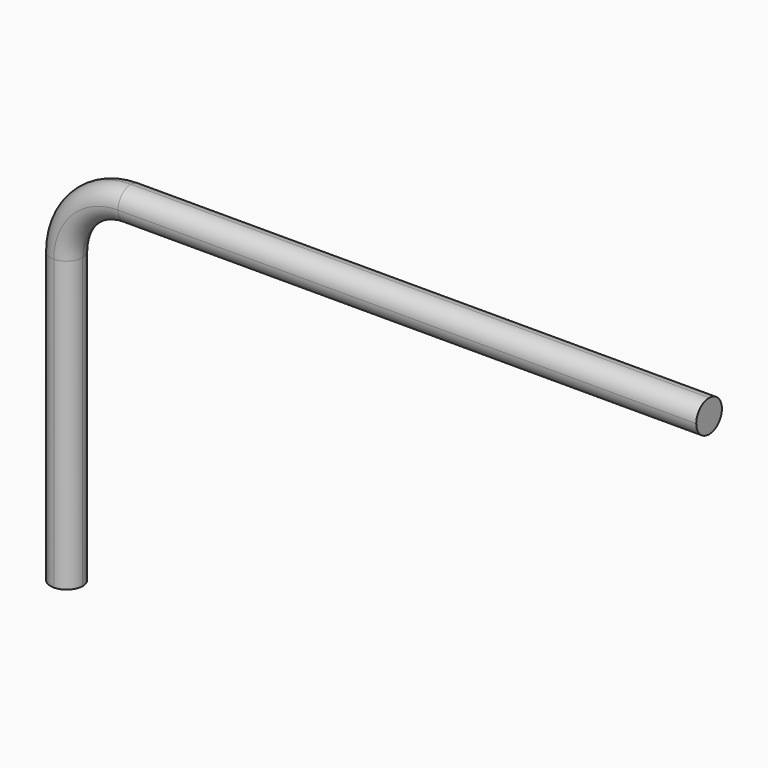
from build123d import *

# Parameters (mm, degrees)
F1_DEPTH = 25.4
F2_R     = 25.39999


# Not quite as in the source:
# - a fillet or chamfer is up to 0.001 mm smaller than in the source, because OpenCascade refuses the exact size


with BuildPart() as f1:
    # F0 (on Front) → F1 (new body, symmetric)
    with BuildSketch(Plane.XZ):
        with BuildLine():
            Line((-50.8, 0), (0, 0))
            Line((0, 0), (0, 457.2))
            ThreePointArc((0, 457.2), (22.3184632736, 511.0815367264), (76.2, 533.4))
            Line((76.2, 533.4), (990.6, 533.4))
            Line((990.6, 533.4), (990.6, 584.2))
            Line((990.6, 584.2), (76.2, 584.2))
            ThreePointArc((76.2, 584.2), (-13.6025612107, 547.0025612107), (-50.8, 457.2))
            Line((-50.8, 457.2), (-50.8, 0))
        make_face()
    extrude(amount=F1_DEPTH, both=True)

    # F2 (radius 25.4 in the source; OpenCascade refuses exactly that, so slightly less here)
    f2_edges = [f1.edges().sort_by_distance(p)[0] for p in [
        (533.4, 25.4, 584.2),
        (533.4, -25.4, 584.2),
        (533.4, 25.4, 533.4),
        (533.4, -25.4, 533.4),
        (-13.602561, -25.4, 547.002561),
        (-13.602561, 25.4, 547.002561),
        (22.318463, -25.4, 511.081537),
        (0, -25.4, 228.6),
        (-50.8, -25.4, 228.6),
        (0, 25.4, 228.6),
        (-50.8, 25.4, 228.6),
        (22.318463, 25.4, 511.081537),
    ]]
    fillet(f2_edges, radius=F2_R)


solid = f1.part
